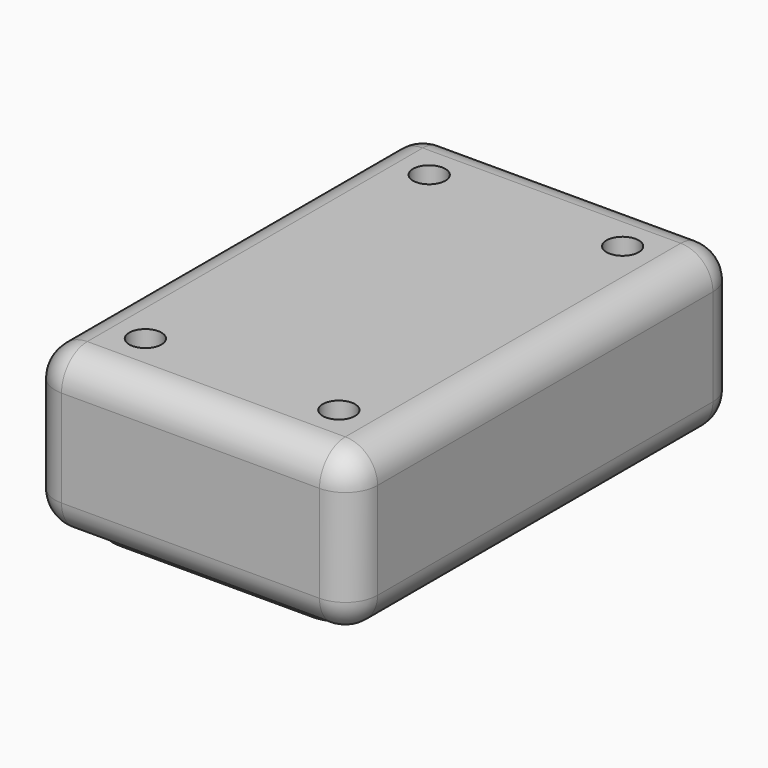
from build123d import *

# Parameters (mm, degrees)
F0_W         = 50.8
F0_H         = 25.4
F1_DEPTH     = 76.2
F2_R         = 5.08
F3_T1_DEPTH  = 15.24
F3_T3_DEPTH  = 40.64
F3_S7_W      = 5.08
F3_S7_H      = 5.08
F3_T8_DEPTH  = 5.08
F3_S13_W     = 5.08
F3_S13_H     = 5.08
F3_T14_DEPTH = 5.08
F3_S19_W     = 5.08
F3_S19_H     = 5.08
F3_T20_DEPTH = 5.08
F3_S25_W     = 5.08
F3_S25_H     = 5.08
F3_T26_DEPTH = 5.08
F3_T30_ANGLE = 90
F3_T32_ANGLE = 90
F3_T34_ANGLE = 90
F3_T36_ANGLE = 90
F5_W         = 40.64
F5_H         = 66.04
F6_DEPTH     = 1.27
F7_R         = 5.08
F8_R         = 2.54
F9_DEPTH     = 101.6
F10_R        = 2.54
F11_DEPTH    = 101.6


# Not quite as in the source:
# - a fillet or chamfer that OpenCascade refuses, or shapes differently, is made with other operations: its cross-section is extruded or revolved along the edge and cut away or added
# - two fillets or chamfers of one size are made in one step


with BuildPart() as f1:
    # F0 (on Front) → F1 (new body)
    with BuildSketch(Plane.XZ):
        Rectangle(F0_W, F0_H)
    extrude(amount=F1_DEPTH)

    # F2
    f2_edges = [f1.edges().sort_by_distance(p)[0] for p in [
        (25.4, -38.1, 12.7),
        (0, 0, 12.7),
        (-25.4, -38.1, 12.7),
        (25.4, -38.1, -12.7),
        (-25.4, -38.1, -12.7),
        (0, 0, -12.7),
    ]]
    fillet(f2_edges, radius=F2_R)

    # F3: fillet of radius 5.08 on 12 edges, made by hand

    # F3_s2 → F3_t1 (cut)
    with BuildSketch(Plane.XY.offset(-7.62)):
        with BuildLine():
            ThreePointArc((25.4, -5.08), (23.9121024484, -1.4878975516), (20.32, 0))
            Line((20.32, 0), (25.4, 0))
            Line((25.4, 0), (25.4, -5.08))
        make_face()
        with BuildLine():
            ThreePointArc((25.4, -71.12), (23.9121024484, -74.7121024484), (20.32, -76.2))
            Line((20.32, -76.2), (25.4, -76.2))
            Line((25.4, -76.2), (25.4, -71.12))
        make_face()
        with BuildLine():
            ThreePointArc((-20.32, 0), (-23.9121024484, -1.4878975516), (-25.4, -5.08))
            Line((-25.4, -5.08), (-25.4, 0))
            Line((-25.4, 0), (-20.32, 0))
        make_face()
        with BuildLine():
            ThreePointArc((-20.32, -76.2), (-23.9121024484, -74.7121024484), (-25.4, -71.12))
            Line((-25.4, -71.12), (-25.4, -76.2))
            Line((-25.4, -76.2), (-20.32, -76.2))
        make_face()
    extrude(amount=F3_T1_DEPTH, mode=Mode.SUBTRACT)

    # F3_s4 → F3_t3 (cut)
    with BuildSketch(Plane.YZ.offset(-20.32)):
        with BuildLine():
            ThreePointArc((-76.2, -7.62), (-74.7121024484, -11.2121024484), (-71.12, -12.7))
            Line((-71.12, -12.7), (-76.2, -12.7))
            Line((-76.2, -12.7), (-76.2, -7.62))
        make_face()
        with BuildLine():
            ThreePointArc((-76.2, 7.62), (-74.7121024484, 11.2121024484), (-71.12, 12.7))
            Line((-71.12, 12.7), (-76.2, 12.7))
            Line((-76.2, 12.7), (-76.2, 7.62))
        make_face()
    extrude(amount=F3_T3_DEPTH, mode=Mode.SUBTRACT)


with BuildPart() as f3_tool6:
    # F3_s7 → F3_t8 (new body)
    with BuildSketch(Plane.YZ.offset(20.32)):
        with Locations((-2.54, 10.16)):
            Rectangle(F3_S7_W, F3_S7_H)
    extrude(amount=F3_T8_DEPTH)

    # F3_s9 → F3_t10 (revolve, cut)
    with BuildSketch(Plane(origin=(20.32, -5.08, 7.62), x_dir=(0, -0.7071067812, -0.7071067812), z_dir=(0, -0.7071067812, 0.7071067812))):
        with BuildLine():
            ThreePointArc((0, -5.08), (5.08, 0), (0, 5.08))
            Line((0, 5.08), (0, -5.08))
        make_face()
    revolve(axis=Axis((20.32, -5.08, 7.62), (1, 0, 0)), mode=Mode.SUBTRACT)


with BuildPart() as f1_1:
    add(f1.part)

    # F3_t5: cut F3_tool6
    add(f3_tool6.part, mode=Mode.SUBTRACT)


with BuildPart() as f3_tool12:
    # F3_s13 → F3_t14 (new body)
    with BuildSketch(Plane.XZ.offset(5.08)):
        with Locations((-22.86, 10.16)):
            Rectangle(F3_S13_W, F3_S13_H)
    extrude(amount=-F3_T14_DEPTH)

    # F3_s15 → F3_t16 (revolve, cut)
    with BuildSketch(Plane(origin=(-20.32, -5.08, 7.62), x_dir=(0.7071067812, 0, -0.7071067812), z_dir=(0.7071067812, 0, 0.7071067812))):
        with BuildLine():
            ThreePointArc((0, -5.08), (5.08, 0), (0, 5.08))
            Line((0, 5.08), (0, -5.08))
        make_face()
    revolve(axis=Axis((-20.32, -5.08, 7.62), (0, 1, 0)), mode=Mode.SUBTRACT)


with BuildPart() as f1_2:
    add(f1_1.part)

    # F3_t11: cut F3_tool12
    add(f3_tool12.part, mode=Mode.SUBTRACT)


with BuildPart() as f3_tool18:
    # F3_s19 → F3_t20 (new body)
    with BuildSketch(Plane.XZ.offset(5.08)):
        with Locations((-22.86, -10.16)):
            Rectangle(F3_S19_W, F3_S19_H)
    extrude(amount=-F3_T20_DEPTH)

    # F3_s21 → F3_t22 (revolve, cut)
    with BuildSketch(Plane(origin=(-20.32, -5.08, -7.62), x_dir=(0.7071067812, 0, 0.7071067812), z_dir=(-0.7071067812, 0, 0.7071067812))):
        with BuildLine():
            ThreePointArc((0, -5.08), (5.08, 0), (0, 5.08))
            Line((0, 5.08), (0, -5.08))
        make_face()
    revolve(axis=Axis((-20.32, -5.08, -7.62), (0, 1, 0)), mode=Mode.SUBTRACT)


with BuildPart() as f1_3:
    add(f1_2.part)

    # F3_t17: cut F3_tool18
    add(f3_tool18.part, mode=Mode.SUBTRACT)


with BuildPart() as f3_tool24:
    # F3_s25 → F3_t26 (new body)
    with BuildSketch(Plane.YZ.offset(20.32)):
        with Locations((-2.54, -10.16)):
            Rectangle(F3_S25_W, F3_S25_H)
    extrude(amount=F3_T26_DEPTH)

    # F3_s27 → F3_t28 (revolve, cut)
    with BuildSketch(Plane(origin=(20.32, -5.08, -7.62), x_dir=(0, -0.7071067812, 0.7071067812), z_dir=(0, 0.7071067812, 0.7071067812))):
        with BuildLine():
            ThreePointArc((0, -5.08), (5.08, 0), (0, 5.08))
            Line((0, 5.08), (0, -5.08))
        make_face()
    revolve(axis=Axis((20.32, -5.08, -7.62), (1, 0, 0)), mode=Mode.SUBTRACT)


with BuildPart() as f1_4:
    add(f1_3.part)

    # F3_t23: cut F3_tool24
    add(f3_tool24.part, mode=Mode.SUBTRACT)

    # F3_s29 → F3_t30 (revolve, cut)
    with BuildSketch(Plane.XY.offset(-7.62)):
        with BuildLine():
            ThreePointArc((25.4, -71.12), (23.9121024484, -74.7121024484), (20.32, -76.2))
            Line((20.32, -76.2), (25.4, -76.2))
            Line((25.4, -76.2), (25.4, -71.12))
        make_face()
    revolve(axis=Axis((20.32, -76.2, -7.62), (0, 1, 0)), revolution_arc=F3_T30_ANGLE, mode=Mode.SUBTRACT)

    # F3_s31 → F3_t32 (revolve, cut)
    with BuildSketch(Plane.XY.offset(7.62)):
        with BuildLine():
            ThreePointArc((25.4, -71.12), (23.9121024484, -74.7121024484), (20.32, -76.2))
            Line((20.32, -76.2), (25.4, -76.2))
            Line((25.4, -76.2), (25.4, -71.12))
        make_face()
    revolve(axis=Axis((20.32, -76.2, 7.62), (0, -1, 0)), revolution_arc=F3_T32_ANGLE, mode=Mode.SUBTRACT)

    # F3_s33 → F3_t34 (revolve, cut)
    with BuildSketch(Plane.XY.offset(-7.62)):
        with BuildLine():
            ThreePointArc((-20.32, -76.2), (-23.9121024484, -74.7121024484), (-25.4, -71.12))
            Line((-25.4, -71.12), (-25.4, -76.2))
            Line((-25.4, -76.2), (-20.32, -76.2))
        make_face()
    revolve(axis=Axis((-20.32, -76.2, -7.62), (0, -1, 0)), revolution_arc=F3_T34_ANGLE, mode=Mode.SUBTRACT)

    # F3_s35 → F3_t36 (revolve, cut)
    with BuildSketch(Plane.YZ.offset(-20.32)):
        with BuildLine():
            ThreePointArc((-76.2, 7.62), (-74.7121024484, 11.2121024484), (-71.12, 12.7))
            Line((-71.12, 12.7), (-76.2, 12.7))
            Line((-76.2, 12.7), (-76.2, 7.62))
        make_face()
    revolve(axis=Axis((-20.32, -76.2, 7.62), (0, -1, 0)), revolution_arc=F3_T36_ANGLE, mode=Mode.SUBTRACT)


with BuildPart() as f6:
    # F5 (on face) → F6 (new body)
    with BuildSketch(Plane(origin=(0, 0, -12.7), x_dir=(1, 0, 0), z_dir=(0, 0, -1))):
        with Locations((0, 38.1)):
            Rectangle(F5_W, F5_H)
    extrude(amount=F6_DEPTH)

    # F7
    f7_edges = [f6.edges().sort_by_distance(p)[0] for p in [
        (-20.32, -5.08, -13.335),
        (20.32, -5.08, -13.335),
        (20.32, -71.12, -13.335),
        (-20.32, -71.12, -13.335),
    ]]
    fillet(f7_edges, radius=F7_R)


with BuildPart() as f9_tool:
    # F8 (on face) → F9 (new body)
    with BuildSketch(Plane(origin=(0, 0, -13.97), x_dir=(1, 0, 0), z_dir=(0, 0, -1))):
        with Locations((15.24, 10.16)):
            Circle(F8_R)
        with Locations((15.24, 66.04)):
            Circle(F8_R)
        with Locations((-15.24, 66.04)):
            Circle(F8_R)
        with Locations((-15.24, 10.16)):
            Circle(F8_R)
    extrude(amount=-F9_DEPTH)


with BuildPart() as f1_5:
    add(f1_4.part)

    # F9: cut by f9_tool
    add(f9_tool.part, mode=Mode.SUBTRACT)

    # F10 (on face) → F11 (cut)
    with BuildSketch(Plane(origin=(0, 0, -12.7), x_dir=(1, 0, 0), z_dir=(0, 0, -1))):
        with Locations((15.24, 66.04)):
            Circle(F10_R)
        with Locations((-15.24, 66.04)):
            Circle(F10_R)
        with Locations((15.24, 10.16)):
            Circle(F10_R)
        with Locations((-15.24, 10.16)):
            Circle(F10_R)
    extrude(amount=-F11_DEPTH, mode=Mode.SUBTRACT)


with BuildPart() as f6_1:
    add(f6.part)

    # F9: cut by f9_tool
    add(f9_tool.part, mode=Mode.SUBTRACT)


solid = Compound([f1_5.part, f6_1.part])
